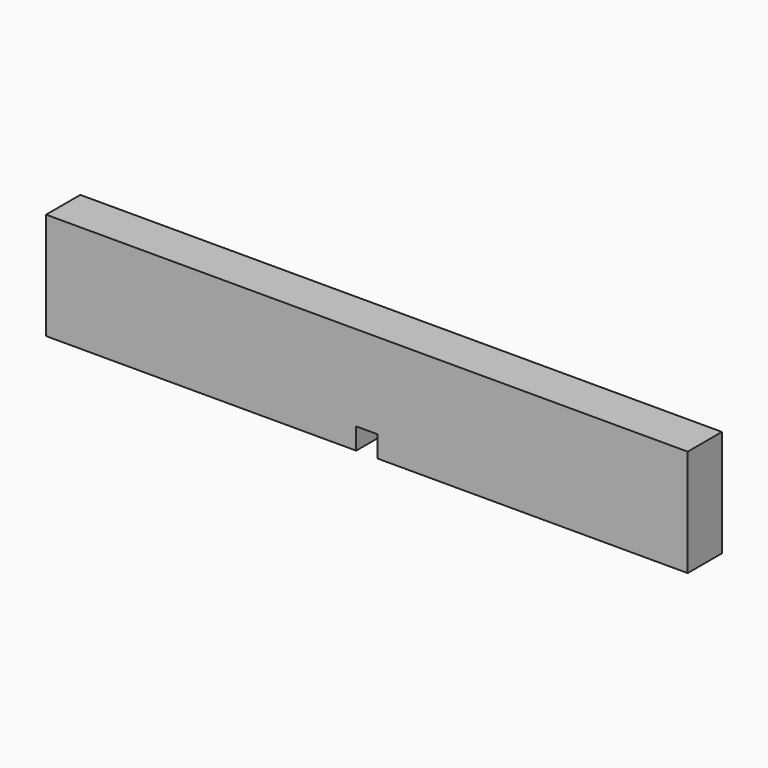
from build123d import *

# Parameters (mm, degrees)
F1_DEPTH = 609.6


# Not quite as in the source:
# - the program builds the solid bodies; features that only make, move or delete a surface that nothing else refers to are left out


with BuildPart() as f1:
    # F0 (on Front) → F1 (new body)
    with BuildSketch(Plane.XZ):
        Polygon((-4597.3245409112, 904.513042295), (-4597.3245409112, -9.886957705), (-177.7245409112, -9.886957705), (-177.7245409112, 294.913042295), (-25.3245409112, 294.913042295), (127.0754590888, 294.913042295), (127.0754590888, -9.886957705), (4546.6754590887, -9.886957705), (4546.6754590888, 1514.113042295), (-4597.3245409112, 1514.113042295), align=None)
    extrude(amount=F1_DEPTH)


solid = f1.part
